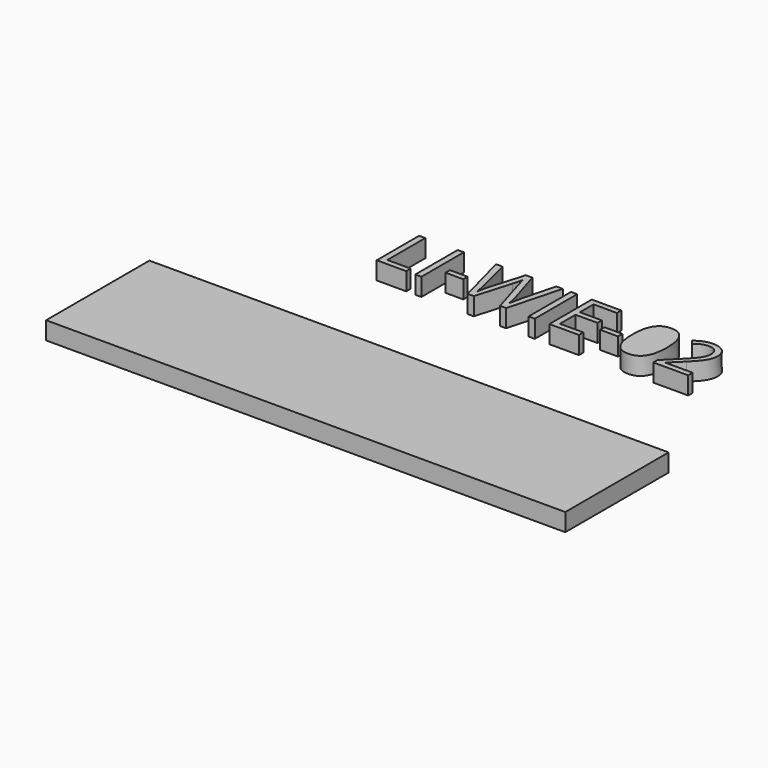
from build123d import *

# Parameters (mm, degrees)
F0_W         = 90.4860690082
F0_H         = 22.507843431
F0_TEXT_SIZE = 12.9464305556
F1_DEPTH     = 3.1


# Not quite as in the source:
# - Text() gives the source's letters only with a copy of the font that has no kerning and outlines rounded to 1/6400 em; it was checked with that copy


with BuildPart() as f1:
    # F0 (on Top) → F1 (new body)
    with BuildSketch(Plane.XY):
        with Locations((-45.2430345041, 24.3266577683)):
            Rectangle(F0_W, F0_H)
        with Locations((-67.6663205052, 54.9814867391)):
            Text('LI-WIE-02', F0_TEXT_SIZE, font='Open Sans', text_align=(TextAlign.LEFT, TextAlign.BOTTOM))
        with BuildLine():
            add(Edge.make_bspline(
                [(-24.0317923336, 62.5460456552), (-24.5061576406, 61.6327154371), (-24.5061576406, 59.6159043021)],
                knots=[0, 0, 0, 1, 1, 1], degree=2))
            add(Edge.make_bspline(
                [(-24.5061576406, 59.6159043021), (-24.5061576406, 57.5990931671), (-24.0317923336, 56.6786828698)],
                knots=[0, 0, 0, 1, 1, 1], degree=2))
            add(Edge.make_bspline(
                [(-24.0317923336, 56.6786828698), (-23.5574270265, 55.7582725725), (-22.521712582, 55.7582725725)],
                knots=[0, 0, 0, 1, 1, 1], degree=2))
            add(Edge.make_bspline(
                [(-22.521712582, 55.7582725725), (-21.4718379792, 55.7582725725), (-21.0015184316, 56.6908201484)],
                knots=[0, 0, 0, 1, 1, 1], degree=2))
            add(Edge.make_bspline(
                [(-21.0015184316, 56.6908201484), (-20.5311988841, 57.6233677244), (-20.5311988841, 59.6159043021)],
                knots=[0, 0, 0, 1, 1, 1], degree=2))
            add(Edge.make_bspline(
                [(-20.5311988841, 59.6159043021), (-20.5311988841, 61.606418), (-21.0015184316, 62.5328969366)],
                knots=[0, 0, 0, 1, 1, 1], degree=2))
            add(Edge.make_bspline(
                [(-21.0015184316, 62.5328969366), (-21.4718379792, 63.4593758733), (-22.521712582, 63.4593758733)],
                knots=[0, 0, 0, 1, 1, 1], degree=2))
            add(Edge.make_bspline(
                [(-22.521712582, 63.4593758733), (-23.5574270265, 63.4593758733), (-24.0317923336, 62.5460456552)],
                knots=[0, 0, 0, 1, 1, 1], degree=2))
        make_face()
    extrude(amount=F1_DEPTH)


solid = f1.part
